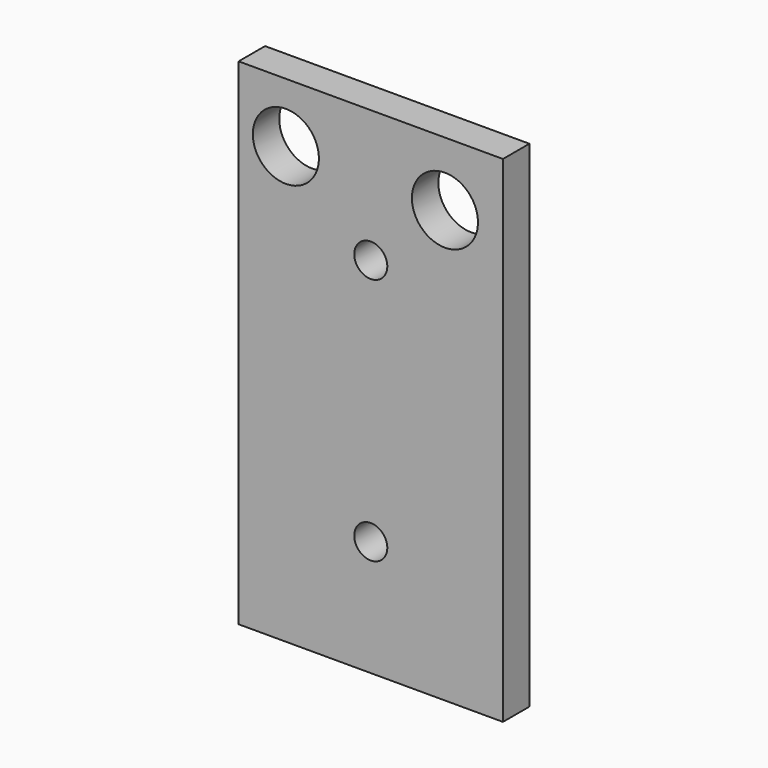
from build123d import *

# Parameters (mm, degrees)
F0_W     = 101.6
F0_H     = 177.8
F1_DEPTH = 12.7
F2_W     = 101.6
F2_H     = 12.7
F3_DEPTH = 12.7
F4_R     = 12.7
F4_R_2   = 6.35
F5_DEPTH = 12.701
F6_R     = 6.35
F7_DEPTH = 12.701


# Not quite as in the source:
# - a feature names something its author has since deleted; it is built from what else it names


with BuildPart() as f1:
    # F0 (on Front) → F1 (new body)
    with BuildSketch(Plane.XZ):
        Rectangle(F0_W, F0_H)
    extrude(amount=F1_DEPTH)

    # F2 (on face) → F3 (join)
    with BuildSketch(Plane(origin=(0, 0, -88.9), x_dir=(1, 0, 0), z_dir=(0, 0, -1))):
        with Locations((0, 6.35)):
            Rectangle(F2_W, F2_H)
    extrude(amount=F3_DEPTH)

    # F4 (on face) → F5 (cut, through all)
    with BuildSketch(Plane(origin=(0, 0, 0), x_dir=(-1, 0, 0), z_dir=(0, 1, 0))):
        with Locations((-28.5075195134, 64.3249601126)):
            Circle(F4_R)
        with Locations((0, 38.1)):
            Circle(F4_R_2)
        with Locations((32.6408334076, 66.04)):
            Circle(F4_R)
    extrude(amount=-F5_DEPTH, mode=Mode.SUBTRACT)

    # F6 (on face) → F7 (cut, through all)
    with BuildSketch(Plane(origin=(0, 0, 0), x_dir=(-1, 0, 0), z_dir=(0, 1, 0))):
        with Locations((0, -57.15)):
            Circle(F6_R)
    extrude(amount=-F7_DEPTH, mode=Mode.SUBTRACT)


solid = f1.part
